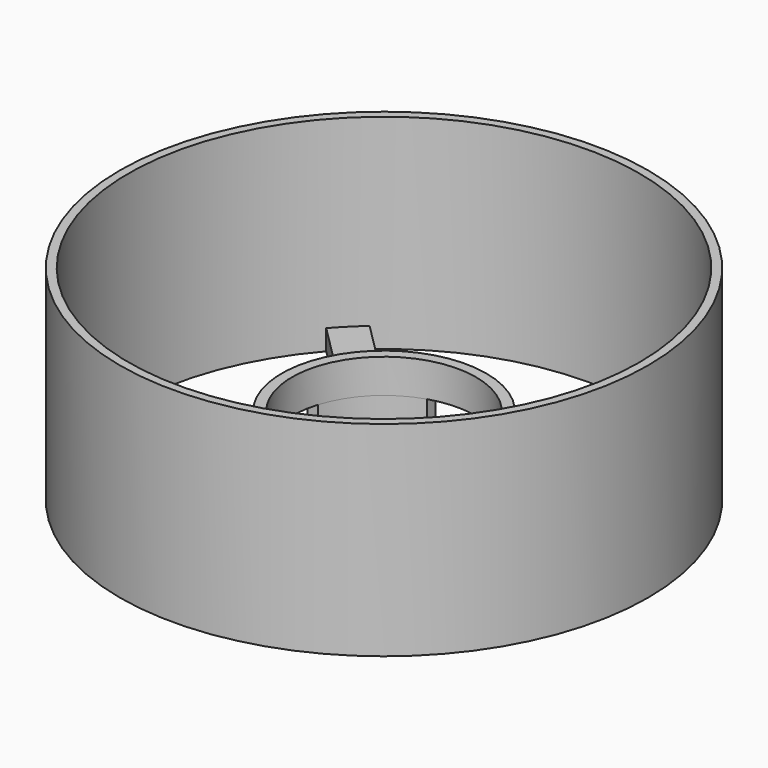
from build123d import *

# Parameters (mm, degrees)
F0_R      = 77.5
F0_R_2    = 75
F1_DEPTH  = 60
F2_R      = 30
F2_R_2    = 1
F3_DEPTH  = 3
F6_DEPTH  = 10
F8_R      = 30
F8_R_2    = 27
F9_DEPTH  = 10
F11_DEPTH = 6


# Not quite as in the source:
# - after a boolean that leaves OpenCascade's solid faulty, fix() repairs it


with BuildPart() as f1:
    # F0 (on Top) → F1 (new body)
    with BuildSketch(Plane.XY):
        Circle(F0_R)
        Circle(F0_R_2, mode=Mode.SUBTRACT)
    extrude(amount=F1_DEPTH)



with BuildPart() as f3:
    # F2 (on Top) → F3 (new body)
    with BuildSketch(Plane.XY):
        Circle(F2_R)
        with Locations((-11.75, -11.75)):
            Circle(F2_R_2, mode=Mode.SUBTRACT)
        with Locations((11.75, -11.75)):
            Circle(F2_R_2, mode=Mode.SUBTRACT)
        with Locations((-11.75, 11.75)):
            Circle(F2_R_2, mode=Mode.SUBTRACT)
        with Locations((11.75, 11.75)):
            Circle(F2_R_2, mode=Mode.SUBTRACT)
    extrude(amount=F3_DEPTH)

    # F5 (on offset) → F6 (join)
    with BuildSketch(Plane.XY.offset(3)):
        with BuildLine():
            ThreePointArc((-8, -25.7875939165), (-19.091883092, -19.091883092), (-25.7875939165, -8))
            Line((-25.7875939165, -8), (-28.9136645896, -8))
            ThreePointArc((-28.9136645896, -8), (-21.2132034356, -21.2132034356), (-8, -28.9136645896))
            Line((-8, -28.9136645896), (-8, -25.7875939165))
        make_face()
        with BuildLine():
            ThreePointArc((-8, 28.9136645896), (-21.2132034356, 21.2132034356), (-28.9136645896, 8))
            Line((-28.9136645896, 8), (-25.7875939165, 8))
            ThreePointArc((-25.7875939165, 8), (-19.091883092, 19.091883092), (-8, 25.7875939165))
            Line((-8, 25.7875939165), (-8, 28.9136645896))
        make_face()
        with BuildLine():
            ThreePointArc((28.9136645896, 8), (21.2132034356, 21.2132034356), (8, 28.9136645896))
            Line((8, 28.9136645896), (8, 25.7875939165))
            ThreePointArc((8, 25.7875939165), (19.091883092, 19.091883092), (25.7875939165, 8))
            Line((25.7875939165, 8), (28.9136645896, 8))
        make_face()
        with BuildLine():
            ThreePointArc((8, -28.9136645896), (21.2132034356, -21.2132034356), (28.9136645896, -8))
            Line((28.9136645896, -8), (25.7875939165, -8))
            ThreePointArc((25.7875939165, -8), (19.091883092, -19.091883092), (8, -25.7875939165))
            Line((8, -25.7875939165), (8, -28.9136645896))
        make_face()
    extrude(amount=F6_DEPTH)

    # F8 (on offset) → F9 (join)
    with BuildSketch(Plane.XY.offset(13)):
        Circle(F8_R)
        Circle(F8_R_2, mode=Mode.SUBTRACT)
    extrude(amount=F9_DEPTH)

    add(f3.part.fix(), mode=Mode.REPLACE)


with BuildPart() as f1_1:
    add(f1.part)

    add(f3.part)  # F11 merges F3
    # F10 (on Top) → F11 (join)
    with BuildSketch(Plane.XY):
        with BuildLine():
            ThreePointArc((-17.3809667574, -24.4520345693), (-21.2132034356, -21.2132034356), (-24.4520345693, -17.3809667574))
            Line((-24.4520345693, -17.3809667574), (-56.4505601272, -49.3794923154))
            ThreePointArc((-56.4505601272, -49.3794923154), (-53.033008589, -53.033008589), (-49.3794923154, -56.4505601272))
            Line((-49.3794923154, -56.4505601272), (-17.3809667574, -24.4520345693))
        make_face()
        with BuildLine():
            ThreePointArc((49.3794923154, -56.4505601272), (53.033008589, -53.033008589), (56.4505601272, -49.3794923154))
            Line((56.4505601272, -49.3794923154), (24.4520345693, -17.3809667574))
            ThreePointArc((24.4520345693, -17.3809667574), (21.2132034356, -21.2132034356), (17.3809667574, -24.4520345693))
            Line((17.3809667574, -24.4520345693), (49.3794923154, -56.4505601272))
        make_face()
        with BuildLine():
            ThreePointArc((56.4505601272, 49.3794923154), (53.033008589, 53.033008589), (49.3794923154, 56.4505601272))
            Line((49.3794923154, 56.4505601272), (17.3809667574, 24.4520345693))
            ThreePointArc((17.3809667574, 24.4520345693), (21.2132034356, 21.2132034356), (24.4520345693, 17.3809667574))
            Line((24.4520345693, 17.3809667574), (56.4505601272, 49.3794923154))
        make_face()
        with BuildLine():
            ThreePointArc((-49.3794923154, 56.4505601272), (-53.033008589, 53.033008589), (-56.4505601272, 49.3794923154))
            Line((-56.4505601272, 49.3794923154), (-24.4520345693, 17.3809667574))
            ThreePointArc((-24.4520345693, 17.3809667574), (-21.2132034356, 21.2132034356), (-17.3809667574, 24.4520345693))
            Line((-17.3809667574, 24.4520345693), (-49.3794923154, 56.4505601272))
        make_face()
    extrude(amount=F11_DEPTH)

    add(f1_1.part.fix(), mode=Mode.REPLACE)


solid = f1_1.part
